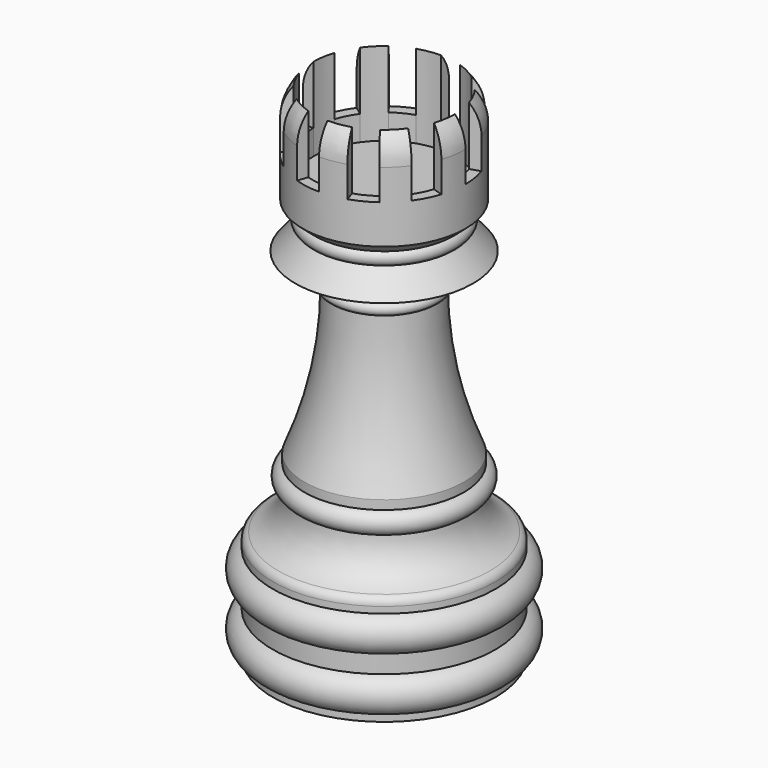
from build123d import *

# Parameters (mm, degrees)
F2_R         = 1
F6_DEPTH     = 7
F7_DEPTH     = 10
F8_T2_ANGLE  = 115.3103509804
F8_T4_ANGLE  = 115.3103509804
F8_T6_ANGLE  = 115.3103509804
F8_T8_ANGLE  = 115.3103509804
F8_T10_ANGLE = 115.3103509804
F8_T12_ANGLE = 115.3103509804
F8_T14_ANGLE = 115.3103509804
F8_T16_ANGLE = 115.3103509804
F8_T18_ANGLE = 115.3103509804
F9_R         = 12.5
F10_DEPTH    = 1
F11_R        = 0.99999


# Not quite as in the source:
# - a fillet or chamfer that OpenCascade refuses, or shapes differently, is made with other operations: its cross-section is extruded or revolved along the edge and cut away or added
# - a fillet or chamfer is up to 0.001 mm smaller than in the source, because OpenCascade refuses the exact size


with BuildPart() as f1:
    # F0 (on Front) → F1 (revolve)
    with BuildSketch(Plane.XZ):
        with BuildLine():
            Line((-21.338325526, 83.376648128), (-21.338325526, 73.376648128))
            Line((-21.338325526, 73.376648128), (-21.338325526, 23.376648128))
            Line((-21.338325526, 23.376648128), (-7.9734302791, 23.376648128))
            Line((-7.9734302791, 23.376648128), (-7.9734302791, 24.2109056562))
            Line((-7.9734302791, 24.2109056562), (-7.9734302791, 28.4109056562))
            Line((-7.9734302791, 28.4109056562), (-7.9734302791, 30.6022372097))
            Line((-7.9734302791, 30.6022372097), (-7.9734302791, 34.8022372097))
            Line((-7.9734302791, 34.8022372097), (-7.9734302791, 36.5691930056))
            Line((-7.9734302791, 36.5691930056), (-11.7825120687, 36.5691930056))
            Line((-11.7825120687, 36.5691930056), (-11.7825120687, 41.1781854928))
            ThreePointArc((-11.7825120687, 41.1781854928), (-10.7919410008, 42.474463582), (-11.7825120687, 43.7707416713))
            Line((-11.7825120687, 43.7707416713), (-11.7825120687, 44.8532998562))
            Line((-11.7825120687, 44.8532998562), (-15.3591325507, 44.8532998562))
            Line((-15.3591325507, 44.8532998562), (-15.3591325507, 62.4988228083))
            ThreePointArc((-15.3591325507, 62.4988228083), (-14.7290810853, 63.195116818), (-15.3591325507, 63.8914108276))
            Line((-15.3591325507, 63.8914108276), (-15.3591325507, 66.1849156022))
            Line((-15.3591325507, 66.1849156022), (-10.6774549931, 66.1849156022))
            Line((-10.6774549931, 66.1849156022), (-12.9833808169, 68.962469697))
            ThreePointArc((-12.9833808169, 68.962469697), (-12.5892002658, 69.7152763605), (-12.9833808169, 70.468083024))
            Line((-12.9833808169, 70.468083024), (-11.5825058892, 71.6823488474))
            Line((-11.5825058892, 71.6823488474), (-11.5825058892, 73.376648128))
            Line((-11.5825058892, 73.376648128), (-11.5825058892, 83.376648128))
            Line((-11.5825058892, 83.376648128), (-21.338325526, 83.376648128))
        make_face()
        with BuildLine():
            Line((-7.9734302791, 34.8022372097), (-7.9734302791, 30.6022372097))
            ThreePointArc((-7.9734302791, 30.6022372097), (-6.5098484578, 32.7022372097), (-7.9734302791, 34.8022372097))
        make_face()
        with BuildLine():
            Line((-7.9734302791, 28.4109056562), (-7.9734302791, 24.2109056562))
            ThreePointArc((-7.9734302791, 24.2109056562), (-6.5098484578, 26.3109056562), (-7.9734302791, 28.4109056562))
        make_face()
    revolve(axis=Axis((-21.338325526, 0, 48.376648128), (0, 0, -1)))

    # F2
    f2_edges = [f1.edges().sort_by_distance(p)[0] for p in [
        (-34.703221, 0, 36.569193),
    ]]
    fillet(f2_edges, radius=F2_R)

    # F3: fillet of radius 45.31 on 1 edges, made by hand

    # F3_s1 → F3_t2 (revolve)
    with BuildSketch(Plane.XZ):
        with BuildLine():
            ThreePointArc((-11.7825120687, 44.8532998562), (-14.455976201, 53.4960203737), (-15.3591325507, 62.4975945148))
            Line((-15.3591325507, 62.4975945148), (-15.3591325507, 44.8532998562))
            Line((-15.3591325507, 44.8532998562), (-11.7825120687, 44.8532998562))
        make_face()
    revolve(axis=Axis((-21.338325526, 0, 44.8532998562), (0, 0, -1)))

    # F4: fillet of radius 5.91 on 1 edges, made by hand

    # F4_s1 → F4_t2 (revolve)
    with BuildSketch(Plane.XZ):
        with BuildLine():
            ThreePointArc((-15.3591325507, 63.8914108276), (-13.2881605646, 65.580647728), (-10.6848344981, 66.1849156022))
            Line((-10.6848344981, 66.1849156022), (-15.3591325507, 66.1849156022))
            Line((-15.3591325507, 66.1849156022), (-15.3591325507, 63.8914108276))
        make_face()
    revolve(axis=Axis((-21.338325526, 0, 66.1849156022), (0, 0, -1)))

    # F5 (on face) → F6 (cut)
    with BuildSketch(Plane.XY.offset(83.376648128)):
        with BuildLine():
            Line((-21.338325526, 9.7558196367), (-21.338325526, 8.5))
            ThreePointArc((-21.338325526, 8.5), (-20.0086325731, 8.3953508951), (-18.7116810738, 8.0839803885))
            Line((-18.7116810738, 8.0839803885), (-18.3236114642, 9.2783358373))
            ThreePointArc((-18.3236114642, 9.2783358373), (-19.8121791001, 9.6357093082), (-21.338325526, 9.7558196367))
        make_face()
        with BuildLine():
            ThreePointArc((-16.3421508815, 6.8766444522), (-15.3279178859, 6.0104076401), (-14.4616810738, 4.9961746445))
            Line((-14.4616810738, 4.9961746445), (-13.4457016458, 5.7343269065))
            ThreePointArc((-13.4457016458, 5.7343269065), (-14.4399193048, 6.8984062212), (-15.6039986195, 7.8926238802))
            Line((-15.6039986195, 7.8926238802), (-16.3421508815, 6.8766444522))
        make_face()
        with BuildLine():
            ThreePointArc((-13.2543451375, 2.6266444522), (-12.9429746309, 1.3296929528), (-12.838325526, 0))
            Line((-12.838325526, 0), (-11.5825058892, 0))
            ThreePointArc((-11.5825058892, 0), (-11.7026162178, 1.5261464259), (-12.0599896887, 3.0147140618))
            Line((-12.0599896887, 3.0147140618), (-13.2543451375, 2.6266444522))
        make_face()
        with BuildLine():
            Line((-12.0599896887, -3.0147140618), (-13.2543451375, -2.6266444522))
            ThreePointArc((-13.2543451375, -2.6266444522), (-13.7647700704, -3.8589192478), (-14.4616810738, -4.9961746445))
            Line((-14.4616810738, -4.9961746445), (-13.4457016458, -5.7343269065))
            ThreePointArc((-13.4457016458, -5.7343269065), (-12.6458265808, -4.4290494323), (-12.0599896887, -3.0147140618))
        make_face()
        with BuildLine():
            ThreePointArc((-16.3421508815, -6.8766444522), (-17.4794062782, -7.5735554556), (-18.7116810738, -8.0839803885))
            Line((-18.7116810738, -8.0839803885), (-18.3236114642, -9.2783358373))
            ThreePointArc((-18.3236114642, -9.2783358373), (-16.9092760937, -8.6924989451), (-15.6039986195, -7.8926238802))
            Line((-15.6039986195, -7.8926238802), (-16.3421508815, -6.8766444522))
        make_face()
        with BuildLine():
            Line((-21.338325526, -9.7558196367), (-21.338325526, -8.5))
            ThreePointArc((-21.338325526, -8.5), (-22.6680184788, -8.3953508951), (-23.9649699782, -8.0839803885))
            Line((-23.9649699782, -8.0839803885), (-24.3530395878, -9.2783358373))
            ThreePointArc((-24.3530395878, -9.2783358373), (-22.8644719519, -9.6357093082), (-21.338325526, -9.7558196367))
        make_face()
        with BuildLine():
            ThreePointArc((-26.3345001705, -6.8766444522), (-27.3487331661, -6.0104076401), (-28.2149699782, -4.9961746445))
            Line((-28.2149699782, -4.9961746445), (-29.2309494062, -5.7343269065))
            ThreePointArc((-29.2309494062, -5.7343269065), (-28.2367317472, -6.8984062212), (-27.0726524325, -7.8926238802))
            Line((-27.0726524325, -7.8926238802), (-26.3345001705, -6.8766444522))
        make_face()
        with BuildLine():
            ThreePointArc((-29.4223059145, -2.6266444522), (-29.733676421, -1.3296929528), (-29.838325526, 0))
            Line((-29.838325526, 0), (-31.0941451627, 0))
            ThreePointArc((-31.0941451627, 0), (-30.9740348342, -1.5261464259), (-30.6166613633, -3.0147140618))
            Line((-30.6166613633, -3.0147140618), (-29.4223059145, -2.6266444522))
        make_face()
        with BuildLine():
            Line((-30.6166613633, 3.0147140618), (-29.4223059145, 2.6266444522))
            ThreePointArc((-29.4223059145, 2.6266444522), (-28.9118809816, 3.8589192478), (-28.2149699782, 4.9961746445))
            Line((-28.2149699782, 4.9961746445), (-29.2309494062, 5.7343269065))
            ThreePointArc((-29.2309494062, 5.7343269065), (-30.0308244711, 4.4290494323), (-30.6166613633, 3.0147140618))
        make_face()
        with BuildLine():
            Line((-27.0726524325, 7.8926238802), (-26.3345001705, 6.8766444522))
            ThreePointArc((-26.3345001705, 6.8766444522), (-25.1972447738, 7.5735554556), (-23.9649699782, 8.0839803885))
            Line((-23.9649699782, 8.0839803885), (-24.3530395878, 9.2783358373))
            ThreePointArc((-24.3530395878, 9.2783358373), (-25.7673749582, 8.6924989451), (-27.0726524325, 7.8926238802))
        make_face()
    extrude(amount=-F6_DEPTH, mode=Mode.SUBTRACT)

    # F5 (on face) → F7 (cut)
    with BuildSketch(Plane.XY.offset(83.376648128)):
        with BuildLine():
            Line((-28.2149699782, -4.9961746445), (-21.338325526, 0))
            Line((-21.338325526, 0), (-29.4223059145, -2.6266444522))
            ThreePointArc((-29.4223059145, -2.6266444522), (-28.9118809816, -3.8589192478), (-28.2149699782, -4.9961746445))
        make_face()
        with BuildLine():
            Line((-23.9649699782, -8.0839803885), (-21.338325526, 0))
            Line((-21.338325526, 0), (-26.3345001705, -6.8766444522))
            ThreePointArc((-26.3345001705, -6.8766444522), (-25.1972447738, -7.5735554556), (-23.9649699782, -8.0839803885))
        make_face()
        with BuildLine():
            Line((-18.7116810738, -8.0839803885), (-21.338325526, 0))
            Line((-21.338325526, 0), (-21.338325526, -8.5))
            ThreePointArc((-21.338325526, -8.5), (-20.0086325731, -8.3953508951), (-18.7116810738, -8.0839803885))
        make_face()
        with BuildLine():
            Line((-14.4616810738, -4.9961746445), (-21.338325526, 0))
            Line((-21.338325526, 0), (-16.3421508815, -6.8766444522))
            ThreePointArc((-16.3421508815, -6.8766444522), (-15.3279178859, -6.0104076401), (-14.4616810738, -4.9961746445))
        make_face()
        with BuildLine():
            ThreePointArc((-13.2543451375, -2.6266444522), (-12.9429746309, -1.3296929528), (-12.838325526, 0))
            Line((-12.838325526, 0), (-21.338325526, 0))
            Line((-21.338325526, 0), (-13.2543451375, -2.6266444522))
        make_face()
        with BuildLine():
            Line((-21.338325526, 0), (-13.2543451375, 2.6266444522))
            ThreePointArc((-13.2543451375, 2.6266444522), (-13.7647700704, 3.8589192478), (-14.4616810738, 4.9961746445))
            Line((-14.4616810738, 4.9961746445), (-21.338325526, 0))
        make_face()
        with BuildLine():
            Line((-18.7116810738, 8.0839803885), (-21.338325526, 0))
            Line((-21.338325526, 0), (-16.3421508815, 6.8766444522))
            ThreePointArc((-16.3421508815, 6.8766444522), (-17.4794062782, 7.5735554556), (-18.7116810738, 8.0839803885))
        make_face()
        with BuildLine():
            Line((-23.9649699782, 8.0839803885), (-21.338325526, 0))
            Line((-21.338325526, 0), (-21.338325526, 8.5))
            ThreePointArc((-21.338325526, 8.5), (-22.6680184788, 8.3953508951), (-23.9649699782, 8.0839803885))
        make_face()
        with BuildLine():
            Line((-28.2149699782, 4.9961746445), (-21.338325526, 0))
            Line((-21.338325526, 0), (-26.3345001705, 6.8766444522))
            ThreePointArc((-26.3345001705, 6.8766444522), (-27.3487331661, 6.0104076401), (-28.2149699782, 4.9961746445))
        make_face()
        with BuildLine():
            Line((-29.838325526, 0), (-21.338325526, 0))
            Line((-21.338325526, 0), (-29.4223059145, 2.6266444522))
            ThreePointArc((-29.4223059145, 2.6266444522), (-29.733676421, 1.3296929528), (-29.838325526, 0))
        make_face()
        with BuildLine():
            Line((-21.338325526, -8.5), (-21.338325526, 0))
            Line((-21.338325526, 0), (-23.9649699782, -8.0839803885))
            ThreePointArc((-23.9649699782, -8.0839803885), (-22.6680184788, -8.3953508951), (-21.338325526, -8.5))
        make_face()
        with BuildLine():
            Line((-26.3345001705, -6.8766444522), (-21.338325526, 0))
            Line((-21.338325526, 0), (-28.2149699782, -4.9961746445))
            ThreePointArc((-28.2149699782, -4.9961746445), (-27.3487331661, -6.0104076401), (-26.3345001705, -6.8766444522))
        make_face()
        with BuildLine():
            Line((-29.4223059145, -2.6266444522), (-21.338325526, 0))
            Line((-21.338325526, 0), (-29.838325526, 0))
            ThreePointArc((-29.838325526, 0), (-29.733676421, -1.3296929528), (-29.4223059145, -2.6266444522))
        make_face()
        with BuildLine():
            Line((-29.4223059145, 2.6266444522), (-21.338325526, 0))
            Line((-21.338325526, 0), (-28.2149699782, 4.9961746445))
            ThreePointArc((-28.2149699782, 4.9961746445), (-28.9118809816, 3.8589192478), (-29.4223059145, 2.6266444522))
        make_face()
        with BuildLine():
            Line((-26.3345001705, 6.8766444522), (-21.338325526, 0))
            Line((-21.338325526, 0), (-23.9649699782, 8.0839803885))
            ThreePointArc((-23.9649699782, 8.0839803885), (-25.1972447738, 7.5735554556), (-26.3345001705, 6.8766444522))
        make_face()
        with BuildLine():
            Line((-21.338325526, 8.5), (-21.338325526, 0))
            Line((-21.338325526, 0), (-18.7116810738, 8.0839803885))
            ThreePointArc((-18.7116810738, 8.0839803885), (-20.0086325731, 8.3953508951), (-21.338325526, 8.5))
        make_face()
        with BuildLine():
            Line((-16.3421508815, 6.8766444522), (-21.338325526, 0))
            Line((-21.338325526, 0), (-14.4616810738, 4.9961746445))
            ThreePointArc((-14.4616810738, 4.9961746445), (-15.3279178859, 6.0104076401), (-16.3421508815, 6.8766444522))
        make_face()
        with BuildLine():
            Line((-21.338325526, 0), (-12.838325526, 0))
            ThreePointArc((-12.838325526, 0), (-12.9429746309, 1.3296929528), (-13.2543451375, 2.6266444522))
            Line((-13.2543451375, 2.6266444522), (-21.338325526, 0))
        make_face()
        with BuildLine():
            ThreePointArc((-14.4616810738, -4.9961746445), (-13.7647700704, -3.8589192478), (-13.2543451375, -2.6266444522))
            Line((-13.2543451375, -2.6266444522), (-21.338325526, 0))
            Line((-21.338325526, 0), (-14.4616810738, -4.9961746445))
        make_face()
        with BuildLine():
            Line((-16.3421508815, -6.8766444522), (-21.338325526, 0))
            Line((-21.338325526, 0), (-18.7116810738, -8.0839803885))
            ThreePointArc((-18.7116810738, -8.0839803885), (-17.4794062782, -7.5735554556), (-16.3421508815, -6.8766444522))
        make_face()
    extrude(amount=-F7_DEPTH, mode=Mode.SUBTRACT)

    # F8: fillet of radius 5 on 9 edges, made by hand

    # F8_s1 → F8_t2 (revolve, cut)
    with BuildSketch(Plane(origin=(-21.1531763194, 1.9790133434, 0), x_dir=(0, 0, 1), z_dir=(0.9956521287, -0.0931495497, 0))):
        with BuildLine():
            ThreePointArc((80.0628718218, 11.74347505), (81.8347491009, 11.4189911614), (83.376648128, 10.4876554133))
            Line((83.376648128, 10.4876554133), (83.376648128, 11.74347505))
            Line((83.376648128, 11.74347505), (80.0628718218, 11.74347505))
        make_face()
    revolve(axis=Axis((-21.338325526, 0, 83.376648128), (0, 0, -1)), revolution_arc=F8_T2_ANGLE, mode=Mode.SUBTRACT)

    # F8_s3 → F8_t4 (revolve, cut)
    with BuildSketch(Plane(origin=(-15.7910546572, -9.3593406545, 0), x_dir=(0, 0, 1), z_dir=(0.8602514242, 0.509870069, 0))):
        with BuildLine():
            ThreePointArc((80.0628718218, -1.123953871), (81.8347491009, -1.4484377595), (83.376648128, -2.3797735077))
            Line((83.376648128, -2.3797735077), (83.376648128, -1.123953871))
            Line((83.376648128, -1.123953871), (80.0628718218, -1.123953871))
        make_face()
    revolve(axis=Axis((-21.338325526, 0, 83.376648128), (0, 0, -1)), revolution_arc=F8_T4_ANGLE, mode=Mode.SUBTRACT)

    # F8_s5 → F8_t6 (revolve, cut)
    with BuildSketch(Plane(origin=(-3.350652484, -7.7634039801, 0), x_dir=(0, 0, 1), z_dir=(0.3962639145, 0.9181366511, 0))):
        with BuildLine():
            ThreePointArc((80.0628718218, -9.8356791019), (81.8347491009, -10.1601629905), (83.376648128, -11.0914987386))
            Line((83.376648128, -11.0914987386), (83.376648128, -9.8356791019))
            Line((83.376648128, -9.8356791019), (80.0628718218, -9.8356791019))
        make_face()
    revolve(axis=Axis((-21.338325526, 0, 83.376648128), (0, 0, -1)), revolution_arc=F8_T6_ANGLE, mode=Mode.SUBTRACT)

    # F8_s7 → F8_t8 (revolve, cut)
    with BuildSketch(Plane(origin=(-1.0241827693, 4.5612931264, 0), x_dir=(0, 0, 1), z_dir=(-0.2190829421, 0.9757062388, 0))):
        with BuildLine():
            ThreePointArc((80.0628718218, -11.0641177052), (81.8347491009, -11.3886015938), (83.376648128, -12.319937342))
            Line((83.376648128, -12.319937342), (83.376648128, -11.0641177052))
            Line((83.376648128, -11.0641177052), (80.0628718218, -11.0641177052))
        make_face()
    revolve(axis=Axis((-21.338325526, 0, 83.376648128), (0, 0, -1)), revolution_arc=F8_T8_ANGLE, mode=Mode.SUBTRACT)

    # F8_s9 → F8_t10 (revolve, cut)
    with BuildSketch(Plane(origin=(-21.1531763194, 1.9790133434, 0), x_dir=(0, 0, 1), z_dir=(-0.9956521287, 0.0931495497, 0))):
        with BuildLine():
            ThreePointArc((80.0628718218, 7.7681642235), (81.8347491009, 7.4436803349), (83.376648128, 6.5123445867))
            Line((83.376648128, 6.5123445867), (83.376648128, 7.7681642235))
            Line((83.376648128, 7.7681642235), (80.0628718218, 7.7681642235))
        make_face()
    revolve(axis=Axis((-21.338325526, 0, 83.376648128), (0, 0, -1)), revolution_arc=F8_T10_ANGLE, mode=Mode.SUBTRACT)

    # F8_s11 → F8_t12 (revolve, cut)
    with BuildSketch(Plane(origin=(-15.7910546572, -9.3593406545, 0), x_dir=(0, 0, 1), z_dir=(-0.8602514242, -0.509870069, 0))):
        with BuildLine():
            ThreePointArc((80.0628718218, 20.6355931445), (81.8347491009, 20.3111092559), (83.376648128, 19.3797735077))
            Line((83.376648128, 19.3797735077), (83.376648128, 20.6355931445))
            Line((83.376648128, 20.6355931445), (80.0628718218, 20.6355931445))
        make_face()
    revolve(axis=Axis((-21.338325526, 0, 83.376648128), (0, 0, -1)), revolution_arc=F8_T12_ANGLE, mode=Mode.SUBTRACT)

    # F8_s13 → F8_t14 (revolve, cut)
    with BuildSketch(Plane(origin=(-3.350652484, -7.7634039801, 0), x_dir=(0, 0, 1), z_dir=(-0.3962639145, -0.9181366511, 0))):
        with BuildLine():
            ThreePointArc((80.0628718218, 29.3473183754), (81.8347491009, 29.0228344868), (83.376648128, 28.0914987386))
            Line((83.376648128, 28.0914987386), (83.376648128, 29.3473183754))
            Line((83.376648128, 29.3473183754), (80.0628718218, 29.3473183754))
        make_face()
    revolve(axis=Axis((-21.338325526, 0, 83.376648128), (0, 0, -1)), revolution_arc=F8_T14_ANGLE, mode=Mode.SUBTRACT)

    # F8_s15 → F8_t16 (revolve, cut)
    with BuildSketch(Plane(origin=(-1.0241827693, 4.5612931264, 0), x_dir=(0, 0, 1), z_dir=(0.2190829421, -0.9757062388, 0))):
        with BuildLine():
            ThreePointArc((80.0628718218, 30.5757569787), (81.8347491009, 30.2512730901), (83.376648128, 29.319937342))
            Line((83.376648128, 29.319937342), (83.376648128, 30.5757569787))
            Line((83.376648128, 30.5757569787), (80.0628718218, 30.5757569787))
        make_face()
    revolve(axis=Axis((-21.338325526, 0, 83.376648128), (0, 0, -1)), revolution_arc=F8_T16_ANGLE, mode=Mode.SUBTRACT)

    # F8_s17 → F8_t18 (revolve, cut)
    with BuildSketch(Plane(origin=(-12.0267475851, 10.5824381649, 0), x_dir=(0, 0, 1), z_dir=(0.7507475611, -0.6605892064, 0))):
        with BuildLine():
            ThreePointArc((80.0628718218, 23.851687161), (81.8347491009, 23.5272032725), (83.376648128, 22.5958675243))
            Line((83.376648128, 22.5958675243), (83.376648128, 23.851687161))
            Line((83.376648128, 23.851687161), (80.0628718218, 23.851687161))
        make_face()
    revolve(axis=Axis((-21.338325526, 0, 83.376648128), (0, 0, -1)), revolution_arc=F8_T18_ANGLE, mode=Mode.SUBTRACT)

    # F9 (on face) → F10 (cut)
    with BuildSketch(Plane(origin=(0, 0, 23.376648128), x_dir=(1, 0, 0), z_dir=(0, 0, -1))):
        with Locations((-21.338325526, 0)):
            Circle(F9_R)
    extrude(amount=-F10_DEPTH, mode=Mode.SUBTRACT)

    # F11 (radius 1 in the source; OpenCascade refuses exactly that, so slightly less here)
    f11_edges = [f1.edges().sort_by_distance(p)[0] for p in [
        (-33.838326, 0, 24.376648),
    ]]
    fillet(f11_edges, radius=F11_R)

    # F12: fillet of radius 5 on 1 edges, made by hand

    # F12_s1 → F12_t2 (revolve)
    with BuildSketch(Plane.XZ):
        with BuildLine():
            ThreePointArc((-8.6083211855, 36.4997280719), (-10.9137387512, 38.3379764388), (-11.7829120687, 41.1555365454))
            Line((-11.7829120687, 41.1555365454), (-12.2830486373, 41.1555365454))
            ThreePointArc((-12.2830486373, 41.1555365454), (-12.2826486373, 38.8623647755), (-12.2826486373, 36.5691930056))
            Line((-12.2826486373, 36.5691930056), (-11.7825120687, 36.069056437))
            ThreePointArc((-11.7825120687, 36.069056437), (-8.9734302791, 36.069056437), (-8.7909986657, 36.0341472246))
            Line((-8.7909986657, 36.0341472246), (-8.6083211855, 36.4997280719))
        make_face()
    revolve(axis=Axis((-21.338325526, 0, 36.5691930056), (0, 0, -1)))


solid = f1.part
